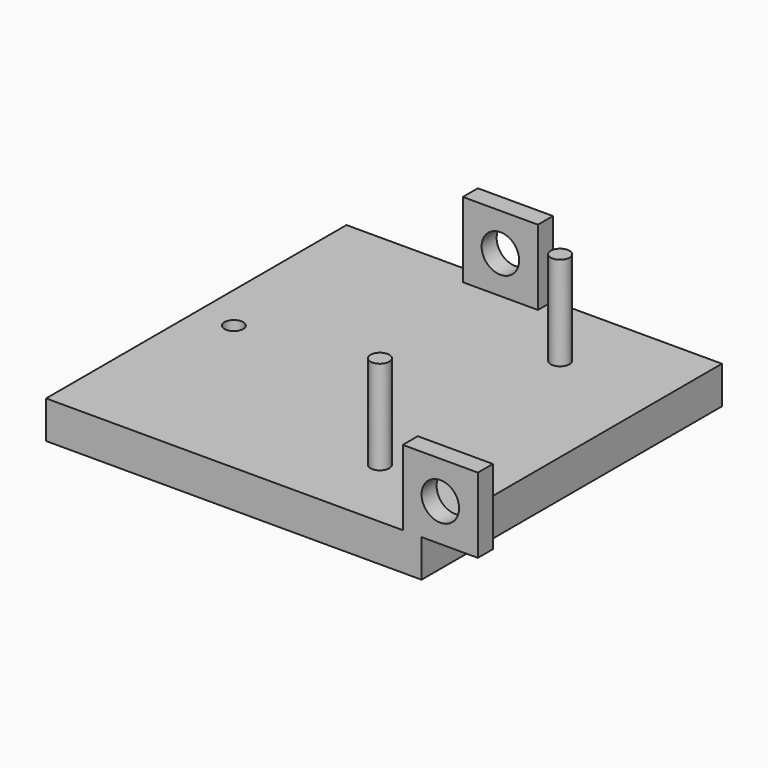
from build123d import *

# Parameters (mm, degrees)
F0_W     = 100
F0_H     = 100
F0_R     = 2.5
F1_DEPTH = 10
F2_R     = 2.5
F3_DEPTH = 25
F4_W     = 20
F4_H     = 20
F5_DEPTH = 5
F6_R     = 5
F7_DEPTH = 25
F8_R     = 5
F9_DEPTH = 5


with BuildPart() as f1:
    # F0 (on Top) → F1 (new body)
    with BuildSketch(Plane.XY):
        with Locations((50, 50)):
            Rectangle(F0_W, F0_H)
        with Locations((10, 50)):
            Circle(F0_R, mode=Mode.SUBTRACT)
    extrude(amount=F1_DEPTH)

    # F2 (on face) → F3 (join)
    with BuildSketch(Plane.XY.offset(10)):
        with Locations((72.9144066572, 20)):
            Circle(F2_R)
        with Locations((72.9144066572, 80)):
            Circle(F2_R)
    extrude(amount=F3_DEPTH)

    # F4 (on face) → F5 (join)
    with BuildSketch(Plane(origin=(0, 100, 0), x_dir=(-1, 0, 0), z_dir=(0, 1, 0))):
        with Locations((-45, 20)):
            Rectangle(F4_W, F4_H)
    extrude(amount=-F5_DEPTH)

    # F6 (on face) → F7 (cut)
    with BuildSketch(Plane(origin=(0, 100, 0), x_dir=(-1, 0, 0), z_dir=(0, 1, 0))):
        with Locations((-45, 20)):
            Circle(F6_R)
    extrude(amount=-F7_DEPTH, mode=Mode.SUBTRACT)

    # F8 (on face) → F9 (join)
    with BuildSketch(Plane.XZ):
        Polygon((95, 30), (95, 10), (100, 10), (115, 10), (115, 30), align=None)
        with Locations((105, 20)):
            Circle(F8_R, mode=Mode.SUBTRACT)
    extrude(amount=-F9_DEPTH)


solid = f1.part
